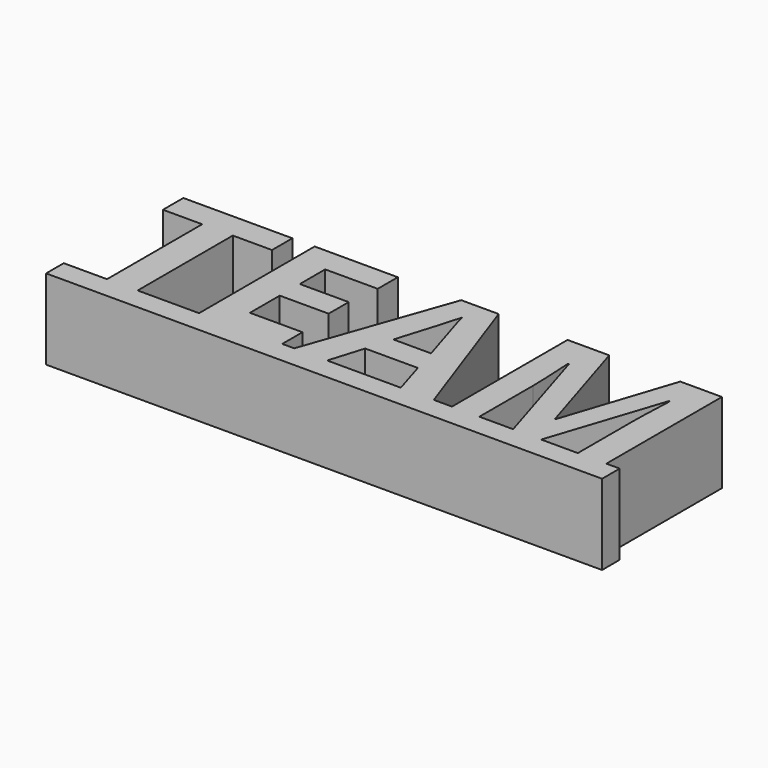
from build123d import *

# Parameters (mm, degrees)
F0_TEXT_SIZE = 31.9807376299
F1_DEPTH     = 12.7


# Not quite as in the source:
# - Text() gives the source's letters only with a copy of the font that has no kerning and outlines rounded to 1/6400 em; it was checked with that copy


with BuildPart() as f1:
    # F0 (on Top) → F1 (new body)
    with BuildSketch(Plane.XY):
        Polygon((-37.0826646799, 0), (-43.9235443385, 0), (-43.9235443385, -3.4888081718), (43.9589843154, -3.4888081718), (43.9589843154, 0), (41.8497933828, 0), (37.3375111829, 0), (31.5459994777, 0), (27.1086721316, 0), (21.7718865396, 0), (17.444492979, 0), (14.5712235826, 0), (9.3543657567, 0), (-2.2786275561, 0), (-7.495485382, 0), (-9.3843476983, 0), (-22.5314290583, 0), (-32.2405811231, 0), align=None)
        with Locations((-43.9235443385, 0)):
            Text('TEAM', F0_TEXT_SIZE, font='Open Sans', font_style=FontStyle.BOLD, text_align=(TextAlign.LEFT, TextAlign.BOTTOM))
    extrude(amount=F1_DEPTH)


solid = f1.part
